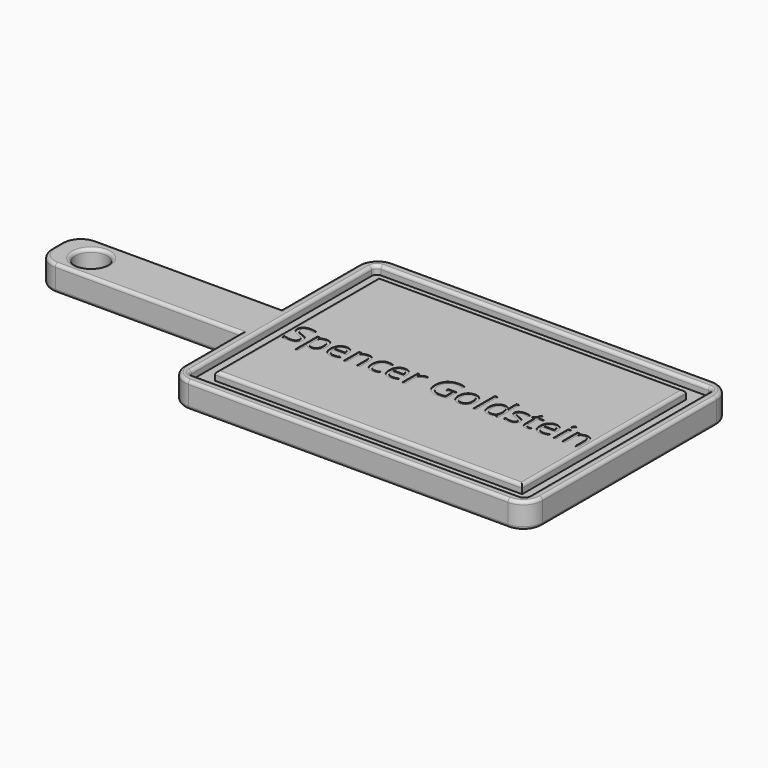
from build123d import *

# Parameters (mm, degrees)
F0_W         = 203.2
F0_H         = 50.8
F1_DEPTH     = 25.4
F2_R         = 15.875
F3_DEPTH     = 25.4
F5_DEPTH     = 8.382
F6_R         = 5.08
F7_R         = 19.05
F8_R         = 3.175
F9_TEXT_SIZE = 35.1867953725
F10_DEPTH    = 0.508


# Not quite as in the source:
# - Text() gives the source's letters only with a copy of the font that has no kerning and outlines rounded to 1/6400 em; it was checked with that copy


with BuildPart() as f1:
    # F0 (on Top) → F1 (new body)
    with BuildSketch(Plane.XY):
        with Locations((-101.6, 114.3)):
            Rectangle(F0_W, F0_H)
        Polygon((0, 88.9), (0, 0), (355.6, 0), (355.6, 254), (0, 254), (0, 139.7), align=None)
    extrude(amount=F1_DEPTH)

    # F2 (on face) → F3 (cut)
    with BuildSketch(Plane.XY.offset(25.4)):
        with Locations((-168.275, 113.665)):
            Circle(F2_R)
    extrude(amount=-F3_DEPTH, mode=Mode.SUBTRACT)

    # F4 (on face) → F5 (cut)
    with BuildSketch(Plane.XY.offset(25.4)):
        Polygon((10.16, 88.9), (10.16, 10.16), (345.44, 10.16), (345.44, 243.84), (10.16, 243.84), (10.16, 139.7), align=None)
        Polygon((25.4, 88.9), (25.4, 139.7), (25.4, 228.6), (330.2, 228.6), (330.2, 25.4), (25.4, 25.4), align=None, mode=Mode.SUBTRACT)
    extrude(amount=-F5_DEPTH, mode=Mode.SUBTRACT)

    # F6
    f6_edges = [f1.edges().sort_by_distance(p)[0] for p in [
        (10.16, 243.84, 21.209),
        (10.16, 10.16, 21.209),
        (345.44, 243.84, 21.209),
        (345.44, 10.16, 21.209),
    ]]
    fillet(f6_edges, radius=F6_R)

    # F7
    f7_edges = [f1.edges().sort_by_distance(p)[0] for p in [
        (0, 254, 12.7),
        (0, 0, 12.7),
        (355.6, 0, 12.7),
        (355.6, 254, 12.7),
        (-203.2, 88.9, 12.7),
        (-203.2, 139.7, 12.7),
    ]]
    fillet(f7_edges, radius=F7_R)

    # F8
    f8_edges = [f1.edges().sort_by_distance(p)[0] for p in [
        (177.8, 228.6, 25.4),
        (330.2, 127, 25.4),
        (177.8, 25.4, 25.4),
        (25.4, 127, 25.4),
        (-92.075, 88.9, 25.4),
        (-197.620384, 94.479616, 25.4),
        (0, 53.975, 25.4),
        (-203.2, 114.3, 25.4),
        (5.579616, 5.579616, 25.4),
        (-197.620384, 134.120384, 25.4),
        (177.8, 0, 25.4),
        (-92.075, 139.7, 25.4),
        (350.020384, 5.579616, 25.4),
        (0, 187.325, 25.4),
        (355.6, 127, 25.4),
        (5.579616, 248.420384, 25.4),
        (350.020384, 248.420384, 25.4),
        (177.8, 254, 25.4),
        (177.8, 10.16, 25.4),
        (11.647898, 11.647898, 25.4),
        (343.952102, 11.647898, 25.4),
        (10.16, 127, 25.4),
        (345.44, 127, 25.4),
        (11.647898, 242.352102, 25.4),
        (343.952102, 242.352102, 25.4),
        (177.8, 243.84, 25.4),
        (-184.15, 113.665, 25.4),
        (-92.075, 88.9, 0),
        (-197.620384, 94.479616, 0),
        (0, 53.975, 0),
        (-203.2, 114.3, 0),
        (5.579616, 5.579616, 0),
        (-197.620384, 134.120384, 0),
        (177.8, 0, 0),
        (-92.075, 139.7, 0),
        (350.020384, 5.579616, 0),
        (0, 187.325, 0),
        (355.6, 127, 0),
        (5.579616, 248.420384, 0),
        (350.020384, 248.420384, 0),
        (177.8, 254, 0),
        (-184.15, 113.665, 0),
    ]]
    fillet(f8_edges, radius=F8_R)

    # F9 (on face) → F10 (cut)
    with BuildSketch(Plane.XY.offset(25.4)):
        with Locations((28.575, 101.6655073318)):
            Text('Spencer Goldstein', F9_TEXT_SIZE, font='Open Sans', text_align=(TextAlign.LEFT, TextAlign.BOTTOM))
    extrude(amount=-F10_DEPTH, mode=Mode.SUBTRACT)


solid = f1.part
